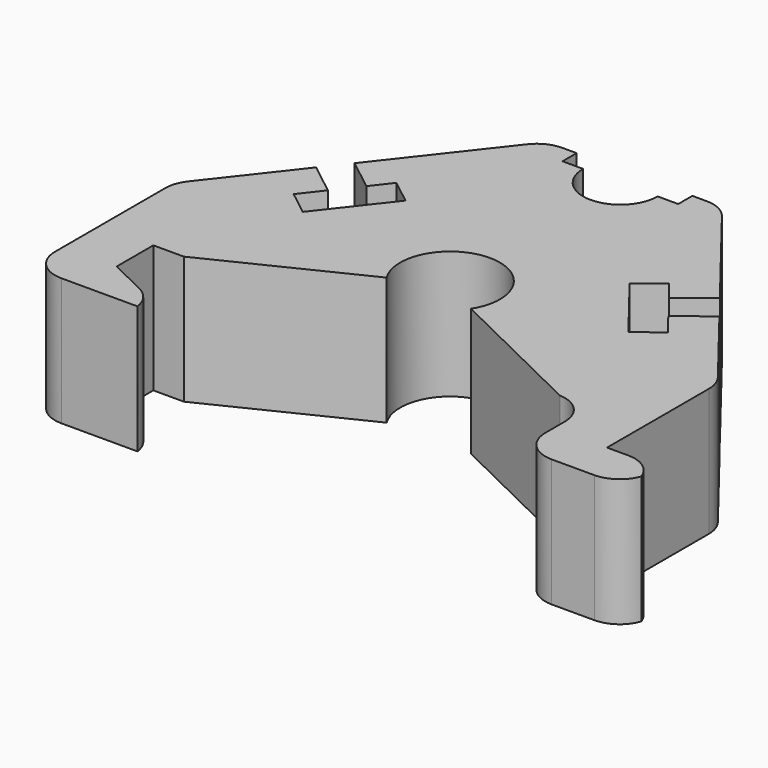
from build123d import *

# Parameters (mm, degrees)
F1_DEPTH    = 12
F3_D        = 5.5
F3_DEPTH    = 7
F3_TIP      = 1.6523667023
F4_T1_DEPTH = 12
F4_T3_DEPTH = 27
F4_T5_DEPTH = 17.1641728771
F4_T7_DEPTH = 19.3168092608
F4_T9_DEPTH = 21.2169428411


# Not quite as in the source:
# - a fillet or chamfer that OpenCascade refuses, or shapes differently, is made with other operations: its cross-section is extruded or revolved along the edge and cut away or added
# - a feature names something its author has since deleted; it is built from what else it names


with BuildPart() as f1:
    # F0 (on Top) → F1 (new body)
    with BuildSketch(Plane.XY):
        with BuildLine():
            Line((5.4365318258, 35.1470746964), (5.4365318258, 33.4868409083))
            Line((5.4365318258, 33.4868409083), (3.5, 33.4868409083))
            ThreePointArc((3.5, 33.4868409083), (0, 29.9868409083), (-3.5, 33.4868409083))
            Line((-3.5, 33.4868409083), (-5.4365318258, 33.4868409083))
            Line((-5.4365318258, 33.4868409083), (-5.4365318258, 35.1470746964))
            Line((-5.4365318258, 35.1470746964), (-8.2365318258, 35.1470746964))
            Line((-8.2365318258, 35.1470746964), (-17.1626134825, 23.7201299491))
            Line((-17.1626134825, 23.7201299491), (-14.2073691514, 21.4116605551))
            Line((-14.2073691514, 21.4116605551), (-12.8128593238, 23.1968768865))
            Line((-12.8128593238, 23.1968768865), (-10.5274703744, 21.4116605551))
            Line((-10.5274703744, 21.4116605551), (-15.298307122, 15.304155604))
            Line((-15.298307122, 15.304155604), (-17.5836960714, 17.0893719354))
            Line((-17.5836960714, 17.0893719354), (-15.9925854827, 19.1262716057))
            Line((-15.9925854827, 19.1262716057), (-18.9478298139, 21.4347409997))
            Line((-18.9478298139, 21.4347409997), (-25.5365714751, 13))
            Line((-25.5365714751, 13), (-25.5365714751, 0))
            Line((-25.5365714751, 0), (-25.5365714751, -4))
            Line((-25.5365714751, -4), (-20.5365714751, -4))
            Line((-20.5365714751, -4), (-15.3852878138, -4))
            Line((-15.3852878138, -4), (-15.3852878138, -2.5156375486))
            Line((-15.3852878138, -2.5156375486), (-20.5365714751, 0))
            Line((-20.5365714751, 0), (-20.5365714751, 4.3))
            Line((-20.5365714751, 4.3), (-17.6668407531, 4.3))
            Line((-17.6668407531, 4.3), (-3.9629505379, 10.990731871))
            ThreePointArc((-3.9629505379, 10.990731871), (0, 18.1703798791), (3.9629505379, 10.990731871))
            Line((3.9629505379, 10.990731871), (17.6668407531, 4.3))
            Line((17.6668407531, 4.3), (20.5365714751, 4.3))
            Line((20.5365714751, 4.3), (20.5365714751, -4))
            Line((20.5365714751, -4), (30.5365714751, -4))
            Line((30.5365714751, -4), (30.5365714751, 0))
            Line((30.5365714751, 0), (25.5365714751, 0))
            Line((25.5365714751, 0), (25.5365714751, 13))
            Line((25.5365714751, 13), (18.9478298139, 21.4347409997))
            Line((18.9478298139, 21.4347409997), (15.9925854827, 19.1262716057))
            Line((15.9925854827, 19.1262716057), (17.5836960714, 17.0893719354))
            Line((17.5836960714, 17.0893719354), (15.298307122, 15.304155604))
            Line((15.298307122, 15.304155604), (10.5274703744, 21.4116605551))
            Line((10.5274703744, 21.4116605551), (12.8128593238, 23.1968768865))
            Line((12.8128593238, 23.1968768865), (14.2073691514, 21.4116605551))
            Line((14.2073691514, 21.4116605551), (17.1626134825, 23.7201299491))
            Line((17.1626134825, 23.7201299491), (8.2365318258, 35.1470746964))
            Line((8.2365318258, 35.1470746964), (5.4365318258, 35.1470746964))
        make_face()
    extrude(amount=F1_DEPTH)

    # F3
    with Locations(Plane(origin=(-22.1660473582, 17.3148600175, 0), x_dir=(-0.6155918384, -0.788065155, 0), z_dir=(-0.788065155, 0.6155918384, 0))):
        with Locations((-15.1406489313, 6.5862988122)):
            Hole(F3_D / 2, depth=F3_DEPTH)
            with Locations((0, 0, -(F3_DEPTH + F3_TIP / 2))):  # 118° drill point
                Cone(0, F3_D / 2, F3_TIP, mode=Mode.SUBTRACT)

    # F4: fillet of radius 3 on 10 edges, made by hand

    # F4_s2 → F4_t1 (join)
    with BuildSketch(Plane.XY):
        with BuildLine():
            ThreePointArc((17.6668407531, 4.3), (19.7034595472, 3.3775817354), (20.5365714751, 1.302829682))
            Line((20.5365714751, 1.302829682), (20.5365714751, 4.3))
            Line((20.5365714751, 4.3), (17.6668407531, 4.3))
        make_face()
    extrude(amount=F4_T1_DEPTH)

    # F4_s4 → F4_t3 (cut)
    with BuildSketch(Plane.XY.offset(-7.5)):
        with BuildLine():
            ThreePointArc((20.5365714751, -1), (21.4152511315, -3.1213203436), (23.5365714751, -4))
            Line((23.5365714751, -4), (20.5365714751, -4))
            Line((20.5365714751, -4), (20.5365714751, -1))
        make_face()
        with BuildLine():
            ThreePointArc((-25.5365714751, -1), (-24.6578918186, -3.1213203436), (-22.5365714751, -4))
            Line((-22.5365714751, -4), (-25.5365714751, -4))
            Line((-25.5365714751, -4), (-25.5365714751, -1))
        make_face()
        with BuildLine():
            ThreePointArc((30.5365714751, -3), (29.6578918186, -0.8786796564), (27.5365714751, 0))
            Line((27.5365714751, 0), (30.5365714751, 0))
            Line((30.5365714751, 0), (30.5365714751, -3))
        make_face()
        with BuildLine():
            ThreePointArc((27.5365714751, -4), (29.6578918186, -3.1213203436), (30.5365714751, -1))
            Line((30.5365714751, -1), (30.5365714751, -4))
            Line((30.5365714751, -4), (27.5365714751, -4))
        make_face()
    extrude(amount=F4_T3_DEPTH, mode=Mode.SUBTRACT)

    # F4_s6 → F4_t5 (cut)
    with BuildSketch(Plane.XY.offset(-2.5820864386)):
        with BuildLine():
            ThreePointArc((25.5365714751, 11.9671654246), (25.3731703536, 12.9437445573), (24.90076694, 13.8139409398))
            Line((24.90076694, 13.8139409398), (25.5365714751, 13))
            Line((25.5365714751, 13), (25.5365714751, 11.9671654246))
        make_face()
        with BuildLine():
            ThreePointArc((-24.90076694, 13.8139409398), (-25.3731703536, 12.9437445573), (-25.5365714751, 11.9671654246))
            Line((-25.5365714751, 11.9671654246), (-25.5365714751, 13))
            Line((-25.5365714751, 13), (-24.90076694, 13.8139409398))
        make_face()
    extrude(amount=F4_T5_DEPTH, mode=Mode.SUBTRACT)

    # F4_s8 → F4_t7 (cut)
    with BuildSketch(Plane.XY.offset(-3.6584046304)):
        with BuildLine():
            ThreePointArc((9.1373654386, 33.9938502116), (8.088402549, 34.843398726), (6.7731699737, 35.1470746964))
            Line((6.7731699737, 35.1470746964), (8.2365318258, 35.1470746964))
            Line((8.2365318258, 35.1470746964), (9.1373654386, 33.9938502116))
        make_face()
        with BuildLine():
            ThreePointArc((-6.7731699737, 35.1470746964), (-8.088402549, 34.843398726), (-9.1373654386, 33.9938502116))
            Line((-9.1373654386, 33.9938502116), (-8.2365318258, 35.1470746964))
            Line((-8.2365318258, 35.1470746964), (-6.7731699737, 35.1470746964))
        make_face()
    extrude(amount=F4_T7_DEPTH, mode=Mode.SUBTRACT)

    # F4_s10 → F4_t9 (cut)
    with BuildSketch(Plane.XY.offset(-4.6084714206)):
        with BuildLine():
            ThreePointArc((-15.3852878138, -4), (-15.9262171402, -2.6458583956), (-17.0417102945, -1.7067210022))
            Line((-17.0417102945, -1.7067210022), (-15.3852878138, -2.5156375486))
            Line((-15.3852878138, -2.5156375486), (-15.3852878138, -4))
        make_face()
    extrude(amount=F4_T9_DEPTH, mode=Mode.SUBTRACT)


solid = f1.part
